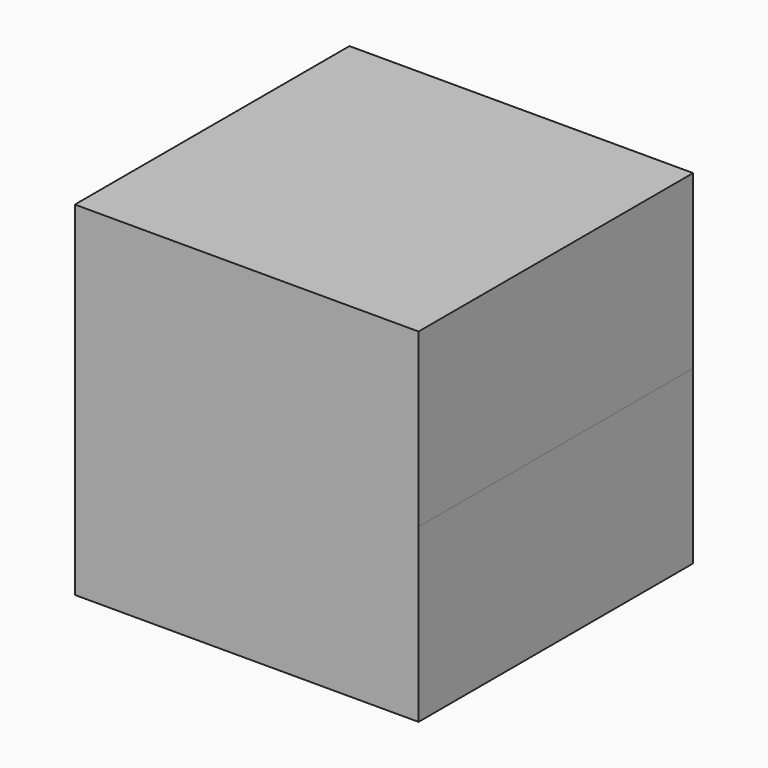
from build123d import *

# Parameters (mm, degrees)
F2_DEPTH = 58.674


# Not quite as in the source:
# - ends of sketch curves that miss each other by under 0.0002 mm in the source are joined
# - the program builds the solid bodies; features that only make, move or delete a surface that nothing else refers to are left out


with BuildPart() as f2:
    # F0 (on Front) → F2 (new body, symmetric)
    with BuildSketch(Plane.XZ):
        with BuildLine():
            Line((-58.7595701218, -58.7595747784), (0, -58.7595747784))
            ThreePointArc((0, -58.7595747784), (41.5492937854, -41.5492937854), (58.7595747784, 0))
            ThreePointArc((58.7595747784, 0), (41.5492937854, 41.5492937854), (0, 58.7595747784))
            Line((0, 58.7595747784), (-58.7595701218, 58.7595747784))
            Line((-58.7595701218, 58.7595747784), (-58.7595701218, -58.7595747784))
        make_face()
        with BuildLine():
            ThreePointArc((0, 58.7595747784), (41.5492937854, 41.5492937854), (58.7595747784, 0))
            Line((58.7595747784, 0), (58.7595701218, 58.7595747784))
            Line((58.7595701218, 58.7595747784), (0, 58.7595747784))
        make_face()
        with BuildLine():
            ThreePointArc((58.7595747784, 0), (41.5492937854, -41.5492937854), (0, -58.7595747784))
            Line((0, -58.7595747784), (58.7595701218, -58.7595747784))
            Line((58.7595701218, -58.7595747784), (58.7595747784, 0))
        make_face()
    extrude(amount=F2_DEPTH, both=True)


solid = f2.part
